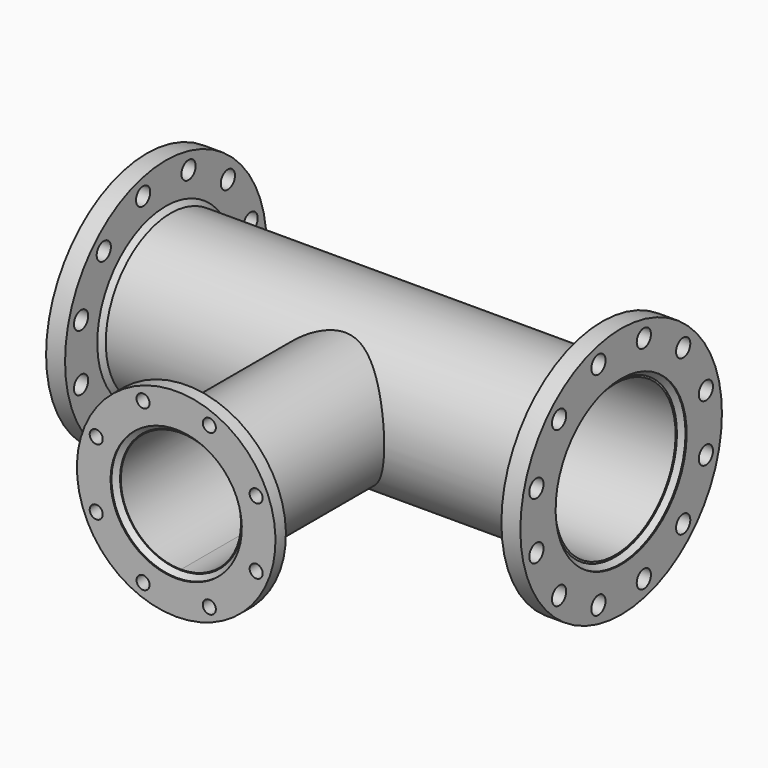
from build123d import *
from build123d import SkipClean  # not in build123d's __all__

# Parameters (mm, degrees)
F6_D      = 30
F6_DEPTH  = 50
F6_TIP    = 9.0129092854
F8_D      = 30
F8_DEPTH  = 50
F8_TIP    = 9.0129092854
F14_D     = 22
F14_DEPTH = 50
F14_TIP   = 6.6094668093
F15_R     = 127.28
F16_DEPTH = 800.001
F17_R     = 101.37
F18_DEPTH = 393


with BuildPart() as f1:
    # F0 (on Front) → F1 (revolve)
    with BuildSketch(Plane.XZ):
        Polygon((-390, 138.15), (-368, 138.15), (-368, 144.55), (-368, 212.5), (-400, 212.5), (-400, 138.15), (-398, 138.15), align=None)
    revolve(axis=Axis((-3.8436072002, 0, 0), (1, 0, 0)))

    # F6
    with Locations(Plane(origin=(-400, 0, 0), x_dir=(0, -1, 0), z_dir=(-1, 0, 0))):
        with Locations((178.6962778635, 47.881523344), (178.6962778635, -47.881523344), (130.8147545195, -130.8147545195), (47.881523344, -178.6962778635), (-47.881523344, -178.6962778635), (-130.8147545195, -130.8147545195), (-178.6962778635, -47.881523344), (-178.6962778635, 47.881523344), (-130.8147545195, 130.8147545195), (-47.881523344, 178.6962778635), (47.881523344, 178.6962778635), (130.8147545195, 130.8147545195)):
            Hole(F6_D / 2, depth=F6_DEPTH)
            with Locations((0, 0, -(F6_DEPTH + F6_TIP / 2))):  # 118° drill point
                Cone(0, F6_D / 2, F6_TIP, mode=Mode.SUBTRACT)


with BuildPart() as f2:
    # F0 (on Front) → F2 (revolve)
    with BuildSketch(Plane.XZ):
        Polygon((368, 212.5), (368, 144.55), (368, 138.15), (390, 138.15), (398, 138.15), (400, 138.15), (400, 212.5), align=None)
    revolve(axis=Axis((-3.8436072002, 0, 0), (1, 0, 0)))

    # F8
    with Locations(Plane.YZ.offset(400)):
        with Locations((-130.8147545195, -130.8147545195), (-178.6962778635, -47.881523344), (-178.6962778635, 47.881523344), (-130.8147545195, 130.8147545195), (-47.881523344, 178.6962778635), (47.881523344, 178.6962778635), (130.8147545195, 130.8147545195), (178.6962778635, 47.881523344), (178.6962778635, -47.881523344), (130.8147545195, -130.8147545195), (47.881523344, -178.6962778635), (-47.881523344, -178.6962778635)):
            Hole(F8_D / 2, depth=F8_DEPTH)
            with Locations((0, 0, -(F8_DEPTH + F8_TIP / 2))):  # 118° drill point
                Cone(0, F8_D / 2, F8_TIP, mode=Mode.SUBTRACT)


with BuildPart() as f3:
    # F0 (on Front) → F3 (revolve)
    with BuildSketch(Plane.XZ):
        Polygon((-360, 136.55), (-368, 136.55), (-390, 136.55), (-390, 130.15), (-390, 127.28), (0, 127.28), (0, 136.55), align=None)
        Polygon((360, 136.55), (0, 136.55), (0, 127.28), (390, 127.28), (390, 130.15), (390, 136.55), (368, 136.55), align=None)
    revolve(axis=Axis((-3.8436072002, 0, 0), (1, 0, 0)))

    # F9 (on Right) → F10 (revolve)
    with BuildSketch(Plane.YZ):
        Polygon((0, -109.55), (0, -101.37), (-428.15, -101.37), (-428.15, -102.7), (-428.15, -109.55), (-416.15, -109.55), (-408.15, -109.55), align=None)
    revolve(axis=Axis((0, -365.8227092559, 0), (0, -1, 0)))

    # F15 (on face) → F16 (cut, through all)
    with BuildSketch(Plane(origin=(-400, 0, 0), x_dir=(0, -1, 0), z_dir=(-1, 0, 0))):
        Circle(F15_R)
    extrude(amount=-F16_DEPTH, mode=Mode.SUBTRACT)

    # F17 (on face) → F18 (cut)
    with BuildSketch(Plane.XZ.offset(438.15)):
        Circle(F17_R)
    with SkipClean():  # cleaning this boolean's faces spoils the solid; the shape is the same uncleaned
        extrude(amount=-F18_DEPTH, mode=Mode.SUBTRACT)


with BuildPart() as f4:
    # F0 (on Front) → F4 (revolve)
    with BuildSketch(Plane.XZ):
        Polygon((-390, 136.55), (-390, 138.15), (-398, 138.15), (-390, 130.15), align=None)
    revolve(axis=Axis((-3.8436072002, 0, 0), (1, 0, 0)))


with BuildPart() as f4b:
    # F0 (on Front) → F4, piece 2 (revolve)
    with BuildSketch(Plane.XZ):
        Polygon((-368, 144.55), (-368, 138.15), (-368, 136.55), (-360, 136.55), align=None)
    revolve(axis=Axis((-3.8436072002, 0, 0), (1, 0, 0)))


with BuildPart() as f4c:
    # F0 (on Front) → F4, piece 3 (revolve)
    with BuildSketch(Plane.XZ):
        Polygon((368, 144.55), (360, 136.55), (368, 136.55), (368, 138.15), align=None)
    revolve(axis=Axis((-3.8436072002, 0, 0), (1, 0, 0)))


with BuildPart() as f4d:
    # F0 (on Front) → F4, piece 4 (revolve)
    with BuildSketch(Plane.XZ):
        Polygon((390, 136.55), (390, 130.15), (398, 138.15), (390, 138.15), align=None)
    revolve(axis=Axis((-3.8436072002, 0, 0), (1, 0, 0)))


with BuildPart() as f11:
    # F9 (on Right) → F11 (revolve)
    with BuildSketch(Plane.YZ):
        Polygon((-428.15, -110.7), (-436.15, -110.7), (-438.15, -110.7), (-438.15, -167.5), (-416.15, -167.5), (-416.15, -117.55), (-416.15, -110.7), align=None)
    revolve(axis=Axis((0, -365.8227092559, 0), (0, -1, 0)))

    # F14
    with Locations(Plane.XZ.offset(438.15)):
        with Locations((-55.8717811253, 134.8864117466), (55.8717811253, 134.8864117466), (134.8864117466, 55.8717811253), (134.8864117466, -55.8717811253), (55.8717811253, -134.8864117466), (-55.8717811253, -134.8864117466), (-134.8864117466, -55.8717811253), (-134.8864117466, 55.8717811253)):
            Hole(F14_D / 2, depth=F14_DEPTH)
            with Locations((0, 0, -(F14_DEPTH + F14_TIP / 2))):  # 118° drill point
                Cone(0, F14_D / 2, F14_TIP, mode=Mode.SUBTRACT)


with BuildPart() as f12:
    # F9 (on Right) → F12 (revolve)
    with BuildSketch(Plane.YZ):
        Polygon((-416.15, -117.55), (-408.15, -109.55), (-416.15, -109.55), (-416.15, -110.7), align=None)
    revolve(axis=Axis((0, -365.8227092559, 0), (0, -1, 0)))


with BuildPart() as f12b:
    # F9 (on Right) → F12, piece 2 (revolve)
    with BuildSketch(Plane.YZ):
        Polygon((-428.15, -109.55), (-428.15, -102.7), (-436.15, -110.7), (-428.15, -110.7), align=None)
    revolve(axis=Axis((0, -365.8227092559, 0), (0, -1, 0)))


solid = Compound([f1.part, f2.part, f3.part, f4.part, f4b.part, f4c.part, f4d.part, f11.part, f12.part, f12b.part])
